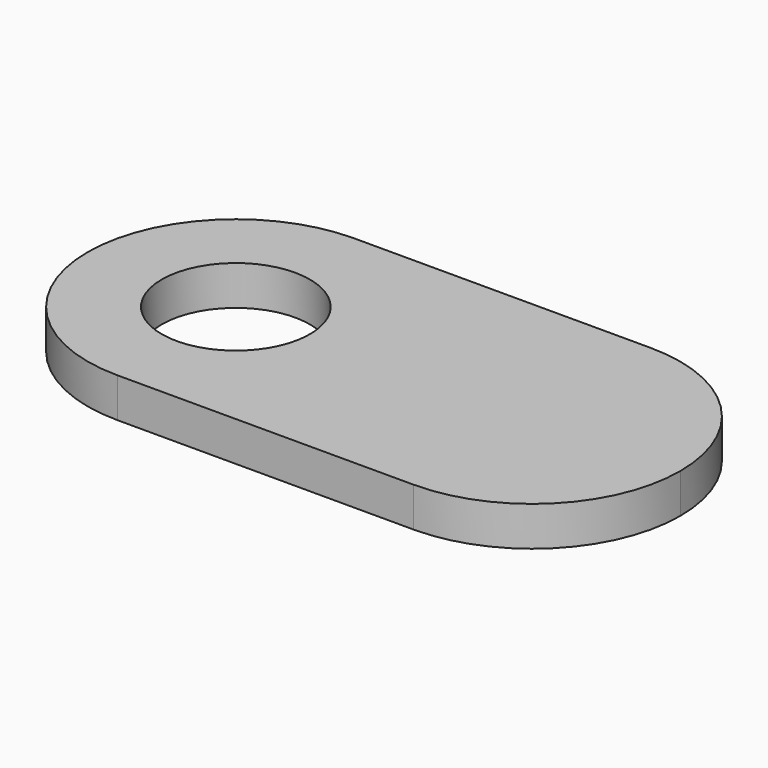
from build123d import *

# Parameters (mm, degrees)
F1_DEPTH = 1.016
F3_D     = 3.81
F4_R     = 1.905
F5_DEPTH = 1.27
F6_R     = 1.26999


# Not quite as in the source:
# - a fillet or chamfer is up to 0.001 mm smaller than in the source, because OpenCascade refuses the exact size


with BuildPart() as f1:
    # F0 (on Top) → F1 (new body)
    with BuildSketch(Plane.XY):
        with BuildLine():
            ThreePointArc((3.81, -3.81), (6.5040768363, -2.6940768363), (7.62, 0))
            ThreePointArc((7.62, 0), (6.5040768363, 2.6940768363), (3.81, 3.81))
            ThreePointArc((3.81, 3.81), (1.1159231637, 2.6940768363), (0, 0))
            ThreePointArc((0, 0), (1.1159231637, -2.6940768363), (3.81, -3.81))
        make_face()
        with BuildLine():
            ThreePointArc((0, 0), (1.1159231637, 2.6940768363), (3.81, 3.81))
            Line((3.81, 3.81), (-3.81, 3.81))
            ThreePointArc((-3.81, 3.81), (-1.1159231637, 2.6940768363), (0, 0))
        make_face()
        with BuildLine():
            Line((-3.81, -3.81), (3.81, -3.81))
            ThreePointArc((3.81, -3.81), (1.1159231637, -2.6940768363), (0, 0))
            ThreePointArc((0, 0), (-1.1159231637, -2.6940768363), (-3.81, -3.81))
        make_face()
        with BuildLine():
            ThreePointArc((-3.81, -3.81), (-1.1159231637, -2.6940768363), (0, 0))
            ThreePointArc((0, 0), (-1.1159231637, 2.6940768363), (-3.81, 3.81))
            ThreePointArc((-3.81, 3.81), (-7.62, 0), (-3.81, -3.81))
        make_face()
    extrude(amount=F1_DEPTH)

    # F3 (through all)
    with Locations(Plane.XY.offset(1.016)):
        with Locations((-3.81, 0)):
            Hole(F3_D / 2)

    # F4 (on face) → F5 (join)
    with BuildSketch(Plane(origin=(0, 0, 0), x_dir=(1, 0, 0), z_dir=(0, 0, -1))):
        with Locations((3.81, 0)):
            Circle(F4_R)
    extrude(amount=F5_DEPTH)

    # F6 (radius 1.27 in the source; OpenCascade refuses exactly that, so slightly less here)
    f6_edges = [f1.edges().sort_by_distance(p)[0] for p in [
        (1.905, 0, -1.27),
    ]]
    fillet(f6_edges, radius=F6_R)


solid = f1.part
